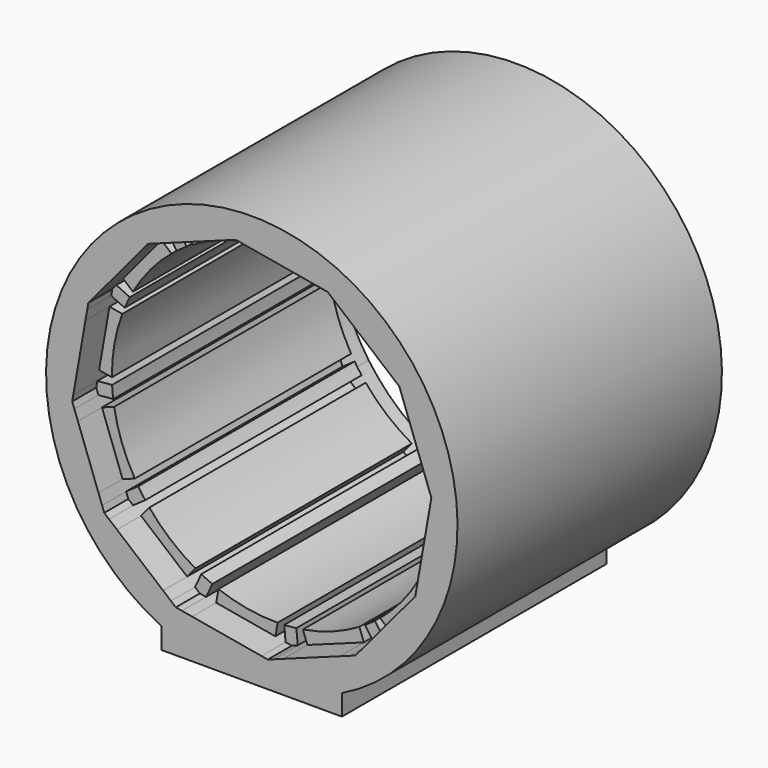
from build123d import *

# Parameters (mm, degrees)
F0_R     = 68.46760183
F1_DEPTH = 100
F3_DEPTH = 90
F4_DEPTH = 10
F2_R     = 54.5558227428
F5_DEPTH = 90
F7_DEPTH = 110


# Not quite as in the source:
# - a feature names something its author has since deleted; it is built from what else it names


with BuildPart() as f1:
    # F0 (on Front) → F1 (new body)
    with BuildSketch(Plane.XZ):
        Circle(F0_R)
        with BuildLine():
            ThreePointArc((-59.7645806946, -5.309886477), (-59.1024517378, 10.3392552235), (-54.4125883665, 25.283793767))
            ThreePointArc((-54.4125883665, 25.283793767), (-46.0145970191, 38.5052835487), (-34.4807869276, 49.1027018896))
            ThreePointArc((-34.4807869276, 49.1027018896), (-20.5971681891, 56.3538522427), (-5.309886477, 59.7645806946))
            ThreePointArc((-5.309886477, 59.7645806946), (10.3392552235, 59.1024517378), (25.283793767, 54.4125883665))
            ThreePointArc((25.283793767, 54.4125883665), (38.5052835487, 46.0145970191), (49.1027018896, 34.4807869276))
            ThreePointArc((49.1027018896, 34.4807869276), (56.3538522427, 20.5971681891), (59.7645806946, 5.309886477))
            ThreePointArc((59.7645806946, 5.309886477), (59.9411162795, 2.657551347), (60, 0))
            ThreePointArc((60, 0), (58.586497173, -12.9469049971), (54.4125883665, -25.283793767))
            ThreePointArc((54.4125883665, -25.283793767), (46.0145970191, -38.5052835487), (34.4807869276, -49.1027018896))
            ThreePointArc((34.4807869276, -49.1027018896), (20.5971681891, -56.3538522427), (5.309886477, -59.7645806946))
            ThreePointArc((5.309886477, -59.7645806946), (-10.3392552235, -59.1024517378), (-25.283793767, -54.4125883665))
            ThreePointArc((-25.283793767, -54.4125883665), (-38.5052835487, -46.0145970191), (-49.1027018896, -34.4807869276))
            ThreePointArc((-49.1027018896, -34.4807869276), (-56.3538522427, -20.5971681891), (-59.7645806946, -5.309886477))
        make_face(mode=Mode.SUBTRACT)
        with BuildLine():
            Line((-54.773548718, 23.2204302764), (-54.4125883665, 25.283793767))
            ThreePointArc((-54.4125883665, 25.283793767), (-59.1024517378, 10.3392552235), (-59.7645806946, -5.309886477))
            Line((-59.7645806946, -5.309886477), (-59.4036203432, -3.2465229864))
            Line((-59.4036203432, -3.2465229864), (-58.8117937345, 0.136545022))
            Line((-58.8117937345, 0.136545022), (-55.3653753266, 19.837362268))
            Line((-55.3653753266, 19.837362268), (-54.773548718, 23.2204302764))
        make_face()
        with BuildLine():
            Line((-59.0454997834, -7.2772918528), (-59.7645806946, -5.309886477))
            ThreePointArc((-59.7645806946, -5.309886477), (-56.3538522427, -20.5971681891), (-49.1027018896, -34.4807869276))
            Line((-49.1027018896, -34.4807869276), (-49.8217828008, -32.5133815518))
            Line((-49.8217828008, -32.5133815518), (-51.0007799272, -29.2876454094))
            Line((-51.0007799272, -29.2876454094), (-57.8665026569, -10.5030279952))
            Line((-57.8665026569, -10.5030279952), (-59.0454997834, -7.2772918528))
        make_face()
        with BuildLine():
            Line((-47.4962568652, -35.825069507), (-49.1027018896, -34.4807869276))
            ThreePointArc((-49.1027018896, -34.4807869276), (-38.5052835487, -46.0145970191), (-25.283793767, -54.4125883665))
            Line((-25.283793767, -54.4125883665), (-26.8902387914, -53.0683057872))
            Line((-26.8902387914, -53.0683057872), (-29.5241483251, -50.8642349052))
            Line((-29.5241483251, -50.8642349052), (-44.8623473315, -38.0291403889))
            Line((-44.8623473315, -38.0291403889), (-47.4962568652, -35.825069507))
        make_face()
        with BuildLine():
            Line((-23.2204302764, -54.773548718), (-25.283793767, -54.4125883665))
            ThreePointArc((-25.283793767, -54.4125883665), (-10.3392552235, -59.1024517378), (5.309886477, -59.7645806946))
            Line((5.309886477, -59.7645806946), (3.2465229864, -59.4036203432))
            Line((3.2465229864, -59.4036203432), (-0.136545022, -58.8117937345))
            Line((-0.136545022, -58.8117937345), (-19.837362268, -55.3653753266))
            Line((-19.837362268, -55.3653753266), (-23.2204302764, -54.773548718))
        make_face()
        with BuildLine():
            Line((7.2772918528, -59.0454997834), (5.309886477, -59.7645806946))
            ThreePointArc((5.309886477, -59.7645806946), (20.5971681891, -56.3538522427), (34.4807869276, -49.1027018896))
            Line((34.4807869276, -49.1027018896), (32.5133815518, -49.8217828008))
            Line((32.5133815518, -49.8217828008), (29.2876454094, -51.0007799272))
            Line((29.2876454094, -51.0007799272), (10.5030279952, -57.8665026569))
            Line((10.5030279952, -57.8665026569), (7.2772918528, -59.0454997834))
        make_face()
        with BuildLine():
            Line((35.825069507, -47.4962568652), (34.4807869276, -49.1027018896))
            ThreePointArc((34.4807869276, -49.1027018896), (46.0145970191, -38.5052835487), (54.4125883665, -25.283793767))
            Line((54.4125883665, -25.283793767), (53.0683057872, -26.8902387914))
            Line((53.0683057872, -26.8902387914), (50.8642349052, -29.5241483251))
            Line((50.8642349052, -29.5241483251), (38.0291403889, -44.8623473315))
            Line((38.0291403889, -44.8623473315), (35.825069507, -47.4962568652))
        make_face()
        with BuildLine():
            ThreePointArc((60, 0), (59.9411162795, 2.657551347), (59.7645806946, 5.309886477))
            Line((59.7645806946, 5.309886477), (59.4036203432, 3.2465229864))
            Line((59.4036203432, 3.2465229864), (58.8117937345, -0.136545022))
            Line((58.8117937345, -0.136545022), (55.3653753266, -19.837362268))
            Line((55.3653753266, -19.837362268), (54.773548718, -23.2204302764))
            Line((54.773548718, -23.2204302764), (54.4125883665, -25.283793767))
            ThreePointArc((54.4125883665, -25.283793767), (58.586497173, -12.9469049971), (60, 0))
        make_face()
        with BuildLine():
            ThreePointArc((-34.4807869276, 49.1027018896), (-46.0145970191, 38.5052835487), (-54.4125883665, 25.283793767))
            Line((-54.4125883665, 25.283793767), (-53.0683057872, 26.8902387914))
            Line((-53.0683057872, 26.8902387914), (-50.8642349052, 29.5241483251))
            Line((-50.8642349052, 29.5241483251), (-38.0291403889, 44.8623473315))
            Line((-38.0291403889, 44.8623473315), (-35.825069507, 47.4962568652))
            Line((-35.825069507, 47.4962568652), (-34.4807869276, 49.1027018896))
        make_face()
        with BuildLine():
            ThreePointArc((-5.309886477, 59.7645806946), (-20.5971681891, 56.3538522427), (-34.4807869276, 49.1027018896))
            Line((-34.4807869276, 49.1027018896), (-32.5133815518, 49.8217828008))
            Line((-32.5133815518, 49.8217828008), (-29.2876454094, 51.0007799272))
            Line((-29.2876454094, 51.0007799272), (-10.5030279952, 57.8665026569))
            Line((-10.5030279952, 57.8665026569), (-7.2772918528, 59.0454997834))
            Line((-7.2772918528, 59.0454997834), (-5.309886477, 59.7645806946))
        make_face()
        with BuildLine():
            ThreePointArc((25.283793767, 54.4125883665), (10.3392552235, 59.1024517378), (-5.309886477, 59.7645806946))
            Line((-5.309886477, 59.7645806946), (-3.2465229864, 59.4036203432))
            Line((-3.2465229864, 59.4036203432), (0.136545022, 58.8117937345))
            Line((0.136545022, 58.8117937345), (19.837362268, 55.3653753266))
            Line((19.837362268, 55.3653753266), (23.2204302764, 54.773548718))
            Line((23.2204302764, 54.773548718), (25.283793767, 54.4125883665))
        make_face()
        with BuildLine():
            ThreePointArc((49.1027018896, 34.4807869276), (38.5052835487, 46.0145970191), (25.283793767, 54.4125883665))
            Line((25.283793767, 54.4125883665), (26.8902387914, 53.0683057872))
            Line((26.8902387914, 53.0683057872), (29.5241483251, 50.8642349052))
            Line((29.5241483251, 50.8642349052), (44.8623473315, 38.0291403889))
            Line((44.8623473315, 38.0291403889), (47.4962568652, 35.825069507))
            Line((47.4962568652, 35.825069507), (49.1027018896, 34.4807869276))
        make_face()
        with BuildLine():
            ThreePointArc((59.7645806946, 5.309886477), (56.3538522427, 20.5971681891), (49.1027018896, 34.4807869276))
            Line((49.1027018896, 34.4807869276), (49.8217828008, 32.5133815518))
            Line((49.8217828008, 32.5133815518), (51.0007799272, 29.2876454094))
            Line((51.0007799272, 29.2876454094), (57.8665026569, 10.5030279952))
            Line((57.8665026569, 10.5030279952), (59.0454997834, 7.2772918528))
            Line((59.0454997834, 7.2772918528), (59.7645806946, 5.309886477))
        make_face()
    extrude(amount=F1_DEPTH)

    # F0 (on Front) → F3 (join)
    with BuildSketch(Plane.XZ):
        Polygon((-38.0291403889, 44.8623473315), (-50.8642349052, 29.5241483251), (-47.0296851536, 26.315374696), (-34.1945906373, 41.6535737024), align=None)
        Polygon((-53.1703483034, -8.7865973127), (-57.8665026569, -10.5030279952), (-51.0007799272, -29.2876454094), (-46.3046255737, -27.571214727), align=None)
        Polygon((19.837362268, 55.3653753266), (0.136545022, 58.8117937345), (-0.7250595799, 53.886589423), (18.975757666, 50.4401710152), align=None)
        Polygon((57.8665026569, 10.5030279952), (51.0007799272, 29.2876454094), (46.3046255737, 27.571214727), (53.1703483034, 8.7865973127), align=None)
        Polygon((34.1945906373, -41.6535737024), (38.0291403889, -44.8623473315), (50.8642349052, -29.5241483251), (47.0296851536, -26.315374696), align=None)
        Polygon((-18.975757666, -50.4401710152), (-19.837362268, -55.3653753266), (-0.136545022, -58.8117937345), (0.7250595799, -53.886589423), align=None)
        Polygon((-49.8217828008, -32.5133815518), (-49.1027018896, -34.4807869276), (-47.4962568652, -35.825069507), (-42.8163366702, -32.5387466598), (-43.979099638, -30.8829026822), (-45.1418626059, -29.2270587046), align=None)
        Polygon((-53.0683057872, 26.8902387914), (-54.4125883665, 25.283793767), (-54.773548718, 23.2204302764), (-49.5875495498, 20.8106619235), (-48.7349280844, 22.645566181), (-47.882306619, 24.4804704385), align=None)
        Polygon((-3.2465229864, 59.4036203432), (-5.309886477, 59.7645806946), (-4.7558284463, 53.5284688632), (-2.7404440131, 53.7075291431), align=None)
        Polygon((-4.7558284463, 53.5284688632), (-5.309886477, 59.7645806946), (-7.2772918528, 59.0454997834), (-6.7712128795, 53.3494085833), align=None)
        Polygon((49.8217828008, 32.5133815518), (49.1027018896, 34.4807869276), (47.4962568652, 35.825069507), (42.8163366702, 32.5387466598), (43.979099638, 30.8829026822), (45.1418626059, 29.2270587046), align=None)
        Polygon((53.0683057872, -26.8902387914), (54.4125883665, -25.283793767), (54.773548718, -23.2204302764), (49.5875495498, -20.8106619235), (48.7349280844, -22.645566181), (47.882306619, -24.4804704385), align=None)
        Polygon((4.7558284463, -53.5284688632), (5.309886477, -59.7645806946), (7.2772918528, -59.0454997834), (6.7712128795, -53.3494085833), align=None)
        Polygon((3.2465229864, -59.4036203432), (5.309886477, -59.7645806946), (4.7558284463, -53.5284688632), (2.7404440131, -53.7075291431), align=None)
        Polygon((-32.5133815518, 49.8217828008), (-34.4807869276, 49.1027018896), (-35.825069507, 47.4962568652), (-32.5387466598, 42.8163366702), (-30.8829026822, 43.979099638), (-29.2270587046, 45.1418626059), align=None)
        Polygon((-10.5030279952, 57.8665026569), (-29.2876454094, 51.0007799272), (-27.571214727, 46.3046255737), (-8.7865973127, 53.1703483034), align=None)
        Polygon((-50.4401710152, 18.975757666), (-55.3653753266, 19.837362268), (-58.8117937345, 0.136545022), (-53.886589423, -0.7250595799), align=None)
        Polygon((-59.4036203432, -3.2465229864), (-59.7645806946, -5.309886477), (-59.0454997834, -7.2772918528), (-53.3494085833, -6.7712128795), (-53.5284688632, -4.7558284463), (-53.7075291431, -2.7404440131), align=None)
        Polygon((-41.6535737024, -34.1945906373), (-44.8623473315, -38.0291403889), (-29.5241483251, -50.8642349052), (-26.315374696, -47.0296851536), align=None)
        Polygon((-26.8902387914, -53.0683057872), (-25.283793767, -54.4125883665), (-23.2204302764, -54.773548718), (-20.8106619235, -49.5875495498), (-22.645566181, -48.7349280844), (-24.4804704385, -47.882306619), align=None)
        Polygon((8.7865973127, -53.1703483034), (10.5030279952, -57.8665026569), (29.2876454094, -51.0007799272), (27.571214727, -46.3046255737), align=None)
        Polygon((32.5133815518, -49.8217828008), (34.4807869276, -49.1027018896), (35.825069507, -47.4962568652), (32.5387466598, -42.8163366702), (30.8829026822, -43.979099638), (29.2270587046, -45.1418626059), align=None)
        Polygon((55.3653753266, -19.837362268), (58.8117937345, -0.136545022), (53.886589423, 0.7250595799), (50.4401710152, -18.975757666), align=None)
        Polygon((59.4036203432, 3.2465229864), (59.7645806946, 5.309886477), (59.0454997834, 7.2772918528), (53.3494085833, 6.7712128795), (53.5284688632, 4.7558284463), (53.7075291431, 2.7404440131), align=None)
        Polygon((44.8623473315, 38.0291403889), (29.5241483251, 50.8642349052), (26.315374696, 47.0296851536), (41.6535737024, 34.1945906373), align=None)
        Polygon((26.8902387914, 53.0683057872), (25.283793767, 54.4125883665), (23.2204302764, 54.773548718), (20.8106619235, 49.5875495498), (22.645566181, 48.7349280844), (24.4804704385, 47.882306619), align=None)
    extrude(amount=F3_DEPTH)

    # F0 (on Front) → F4 (join)
    with BuildSketch(Plane.XZ):
        Circle(F0_R)
        with BuildLine():
            ThreePointArc((-59.7645806946, -5.309886477), (-59.1024517378, 10.3392552235), (-54.4125883665, 25.283793767))
            ThreePointArc((-54.4125883665, 25.283793767), (-46.0145970191, 38.5052835487), (-34.4807869276, 49.1027018896))
            ThreePointArc((-34.4807869276, 49.1027018896), (-20.5971681891, 56.3538522427), (-5.309886477, 59.7645806946))
            ThreePointArc((-5.309886477, 59.7645806946), (10.3392552235, 59.1024517378), (25.283793767, 54.4125883665))
            ThreePointArc((25.283793767, 54.4125883665), (38.5052835487, 46.0145970191), (49.1027018896, 34.4807869276))
            ThreePointArc((49.1027018896, 34.4807869276), (56.3538522427, 20.5971681891), (59.7645806946, 5.309886477))
            ThreePointArc((59.7645806946, 5.309886477), (59.9411162795, 2.657551347), (60, 0))
            ThreePointArc((60, 0), (58.586497173, -12.9469049971), (54.4125883665, -25.283793767))
            ThreePointArc((54.4125883665, -25.283793767), (46.0145970191, -38.5052835487), (34.4807869276, -49.1027018896))
            ThreePointArc((34.4807869276, -49.1027018896), (20.5971681891, -56.3538522427), (5.309886477, -59.7645806946))
            ThreePointArc((5.309886477, -59.7645806946), (-10.3392552235, -59.1024517378), (-25.283793767, -54.4125883665))
            ThreePointArc((-25.283793767, -54.4125883665), (-38.5052835487, -46.0145970191), (-49.1027018896, -34.4807869276))
            ThreePointArc((-49.1027018896, -34.4807869276), (-56.3538522427, -20.5971681891), (-59.7645806946, -5.309886477))
        make_face(mode=Mode.SUBTRACT)
    extrude(amount=-F4_DEPTH)

    # F2 (on Front) → F5 (cut, through all)
    with BuildSketch(Plane.XZ):
        Circle(F2_R)
    extrude(amount=F5_DEPTH, mode=Mode.SUBTRACT)

    # F6 (on face) → F7 (join, through all)
    with BuildSketch(Plane.XZ.offset(100)):
        with BuildLine():
            Line((-30, -68.46760183), (0, -68.46760183))
            ThreePointArc((0, -68.46760183), (-15.3941510863, -66.7145607247), (-30, -61.5452069649))
            Line((-30, -61.5452069649), (-30, -68.46760183))
        make_face()
        with BuildLine():
            ThreePointArc((30, -61.5452069649), (15.3941510863, -66.7145607247), (0, -68.46760183))
            Line((0, -68.46760183), (30, -68.46760183))
            Line((30, -68.46760183), (30, -61.5452069649))
        make_face()
    extrude(amount=-F7_DEPTH)


solid = f1.part
